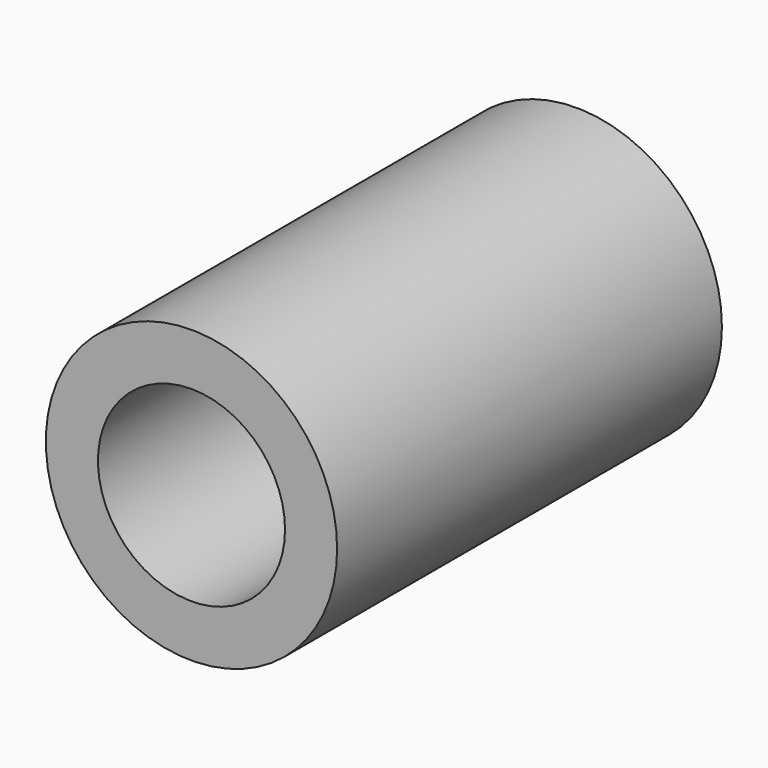
from build123d import *

# Parameters (mm, degrees)
F0_R     = 5.45
F1_DEPTH = 18
F2_E2_W  = 4
F2_E2_H  = 4
F3_DEPTH = 1.5
F4_W     = 1
F4_H     = 1
F5_DEPTH = 2.5


with BuildPart() as f1:
    # F0 (on Front) → F1 (new body)
    with BuildSketch(Plane.XZ):
        Circle(F0_R)
        with BuildLine():
            ThreePointArc((0, 3.5), (2.4748737342, 2.4748737342), (3.5, 0))
            ThreePointArc((3.5, 0), (-2.4748737342, -2.4748737342), (0, 3.5))
        make_face(mode=Mode.SUBTRACT)
    extrude(amount=F1_DEPTH)

    # F2_E2 (on explicit) → F3 (join)
    with BuildSketch(Plane(origin=(2, 0, 3.5), x_dir=(-1, 0, 0), z_dir=(0, 0, 1))):
        with Locations((2, 2)):
            Rectangle(F2_E2_W, F2_E2_H)
    extrude(amount=-F3_DEPTH)

    # F4 (on face) → F5 (cut)
    with BuildSketch(Plane(origin=(0, 0, 2), x_dir=(1, 0, 0), z_dir=(0, 0, -1))):
        with Locations((0, 2)):
            Rectangle(F4_W, F4_H)
    extrude(amount=-F5_DEPTH, mode=Mode.SUBTRACT)


solid = f1.part
